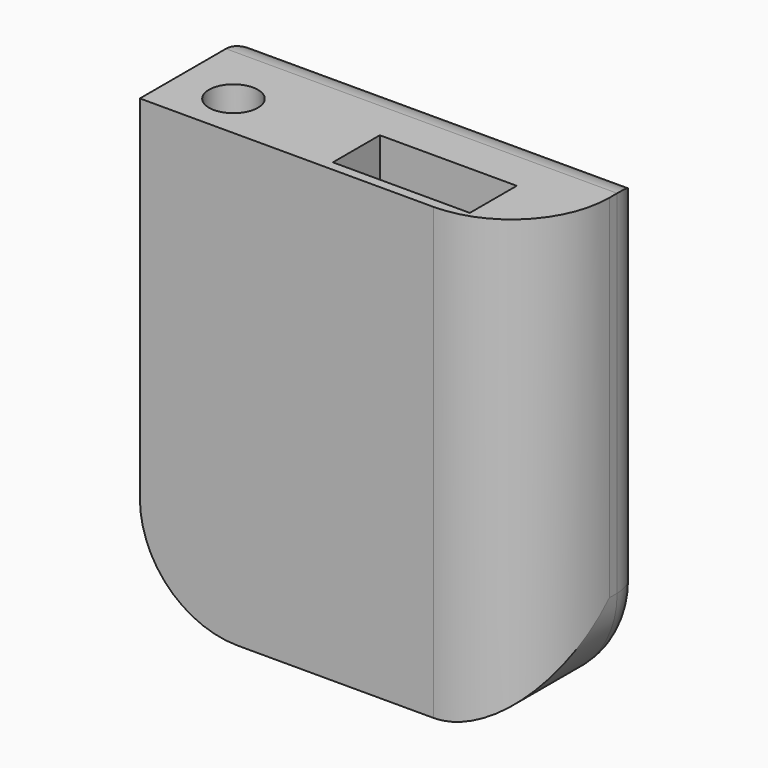
from build123d import *

# Parameters (mm, degrees)
F0_W         = 20
F0_H         = 23
F1_DEPTH     = 7
F2_W         = 15
F2_H         = 3
F3_DEPTH     = 3
F4_W         = 7
F4_H         = 17
F5_DEPTH     = 3
F6_W         = 3
F6_H         = 1
F7_DEPTH     = 3
F8_W         = 2.5268201925
F8_H         = 2
F9_DEPTH     = 3
F10_R        = 1.25
F11_DEPTH    = 5
F12_R        = 2
F13_W        = 5.6845681682
F13_H        = 12.7295220874
F14_DEPTH    = 3
F15_W        = 20
F15_H        = 23
F16_DEPTH    = 0.5
F17_T1_DEPTH = 20
F17_T3_DEPTH = 48
F17_T6_ANGLE = 90
F17_T8_ANGLE = 90
F18_R        = 1.25
F19_DEPTH    = 7


# Not quite as in the source:
# - a fillet or chamfer that OpenCascade refuses, or shapes differently, is made with other operations: its cross-section is extruded or revolved along the edge and cut away or added


with BuildPart() as f1:
    # F0 (on Front) → F1 (new body)
    with BuildSketch(Plane.XZ):
        with Locations((-9.5134219155, 16.3173061975)):
            Rectangle(F0_W, F0_H)
    extrude(amount=F1_DEPTH)

    # F2 (on face) → F3 (cut)
    with BuildSketch(Plane.XZ.offset(7)):
        with Locations((-10.0134219155, 8.3173061975)):
            Rectangle(F2_W, F2_H)
    extrude(amount=-F3_DEPTH, mode=Mode.SUBTRACT)

    # F4 (on face) → F5 (cut)
    with BuildSketch(Plane.XZ.offset(7)):
        with Locations((-6.5459148027, 19.3173061975)):
            Rectangle(F4_W, F4_H)
    extrude(amount=-F5_DEPTH, mode=Mode.SUBTRACT)

    # F6 (on face) → F7 (cut)
    with BuildSketch(Plane.XZ.offset(7)):
        with Locations((-6.5459148027, 10.3173061975)):
            Rectangle(F6_W, F6_H)
    extrude(amount=-F7_DEPTH, mode=Mode.SUBTRACT)

    # F8 (on face) → F9 (cut)
    with BuildSketch(Plane.XZ.offset(7)):
        with Locations((-11.3093248989, 13.8173061975)):
            Rectangle(F8_W, F8_H)
    extrude(amount=-F9_DEPTH, mode=Mode.SUBTRACT)

    # F10 (on face) → F11 (cut)
    with BuildSketch(Plane(origin=(-19.5134219155, 0, 0), x_dir=(0, -1, 0), z_dir=(-1, 0, 0))):
        with Locations((5.55, 8.5673061975)):
            Circle(F10_R)
    extrude(amount=-F11_DEPTH, mode=Mode.SUBTRACT)

    # F12
    f12_edges = [f1.edges().sort_by_distance(p)[0] for p in [
        (0.486578, 0, 16.317306),
        (-19.513422, 0, 16.317306),
        (-9.513422, 0, 27.817306),
        (-9.513422, 0, 4.817306),
    ]]
    fillet(f12_edges, radius=F12_R)

    # F13 (on face) → F14 (cut)
    with BuildSketch(Plane.XZ.offset(7)):
        with Locations((-15.4150190793, 19.1820672412)):
            Rectangle(F13_W, F13_H)
    extrude(amount=-F14_DEPTH, mode=Mode.SUBTRACT)

    # F15 (on face) → F16 (join)
    with BuildSketch(Plane.XZ.offset(7)):
        with Locations((-9.5134219155, 16.3173061975)):
            Rectangle(F15_W, F15_H)
    extrude(amount=F16_DEPTH)

    # F17: fillet of radius 5 on 3 edges, made by hand

    # F17_s2 → F17_t1 (cut)
    with BuildSketch(Plane.XZ):
        with BuildLine():
            ThreePointArc((-19.5134219155, 9.8173061975), (-18.0489558214, 6.2817722916), (-14.5134219155, 4.8173061975))
            Line((-14.5134219155, 4.8173061975), (-19.5134219155, 4.8173061975))
            Line((-19.5134219155, 4.8173061975), (-19.5134219155, 9.8173061975))
        make_face()
        with BuildLine():
            ThreePointArc((0.4865780845, 9.8173061975), (-0.9778880095, 6.2817722916), (-4.5134219155, 4.8173061975))
            Line((-4.5134219155, 4.8173061975), (0.4865780845, 4.8173061975))
            Line((0.4865780845, 4.8173061975), (0.4865780845, 9.8173061975))
        make_face()
    extrude(amount=F17_T1_DEPTH, mode=Mode.SUBTRACT)

    # F17_s4 → F17_t3 (cut)
    with BuildSketch(Plane.XY.offset(-7.6826938025)):
        with BuildLine():
            ThreePointArc((0.4865780845, -2.5), (-0.9778880095, -6.0355339059), (-4.5134219155, -7.5))
            Line((-4.5134219155, -7.5), (0.4865780845, -7.5))
            Line((0.4865780845, -7.5), (0.4865780845, -2.5))
        make_face()
    extrude(amount=F17_T3_DEPTH, mode=Mode.SUBTRACT)

    # F17_s5 → F17_t6 (revolve, cut)
    with BuildSketch(Plane.XY.offset(9.8173061975)):
        with BuildLine():
            ThreePointArc((-1.5134219155, 0), (-0.0992083531, -0.5857864376), (0.4865780845, -2))
            Line((0.4865780845, -2), (0.4865780845, 0))
            Line((0.4865780845, 0), (-1.5134219155, 0))
        make_face()
    revolve(axis=Axis((-4.5134219155, 0, 9.8173061975), (0, 1, 0)), revolution_arc=F17_T6_ANGLE, mode=Mode.SUBTRACT)

    # F17_s7 → F17_t8 (revolve, cut)
    with BuildSketch(Plane.YZ.offset(-14.5134219155)):
        with BuildLine():
            ThreePointArc((0, 6.8173061975), (-0.5857864376, 5.4030926351), (-2, 4.8173061975))
            Line((-2, 4.8173061975), (0, 4.8173061975))
            Line((0, 4.8173061975), (0, 6.8173061975))
        make_face()
    revolve(axis=Axis((-14.5134219155, 0, 9.8173061975), (0, 1, 0)), revolution_arc=F17_T8_ANGLE, mode=Mode.SUBTRACT)

    # F18 (on face) → F19 (cut)
    with BuildSketch(Plane.XY.offset(27.8173061975)):
        with Locations((-16.5796671063, -5.1869219169)):
            Circle(F18_R)
    extrude(amount=-F19_DEPTH, mode=Mode.SUBTRACT)


solid = f1.part
